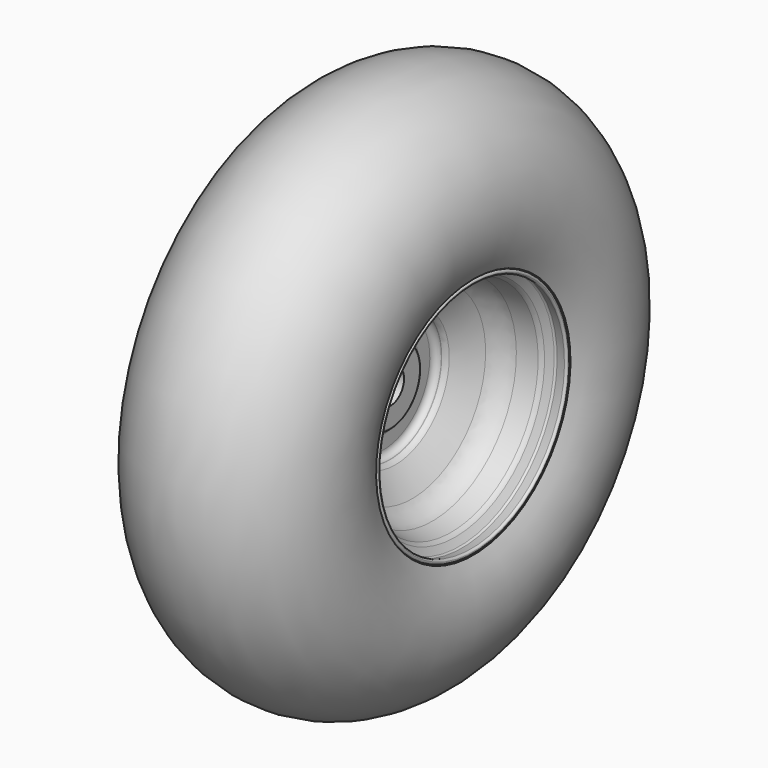
from build123d import *

# Parameters (mm, degrees)
F2_R  = 15
F3_R  = 3
F5_R  = 5
F6_R  = 15
F7_R  = 10
F8_R  = 3
F9_R  = 0.99999
F10_R = 1


# Not quite as in the source:
# - a fillet or chamfer that OpenCascade refuses, or shapes differently, is made with other operations: its cross-section is extruded or revolved along the edge and cut away or added
# - a fillet or chamfer is up to 0.001 mm smaller than in the source, because OpenCascade refuses the exact size


with BuildPart() as f1:
    # F0 (on Front) → F1 (revolve)
    with BuildSketch(Plane.XZ):
        Polygon((-55, 7.9375), (0, 7.9375), (0, 17.9375), (-3.4099393524, 17.9375), (-3.4099393524, 30.2716810256), (1.3420858886, 30.2716810256), (13.6318095028, 47.9688830674), (29.6903830022, 51.0822795331), (32.7981238869, 55.8634183106), (38.7093649285, 54.3856122498), (39.1944348812, 56.3258975744), (31.8988867003, 58.1497794366), (28.4762072553, 52.884119903), (12.4528761376, 49.7775561429), (0.2960184428, 32.2716810256), (-5.4099393524, 32.2716810256), (-5.4099393524, 17.9375), (-9.8811367593, 17.9375), (-5.8835780754, 22.3348141701), (-5.8835780754, 33.0104142308), (-12.7767843909, 37.2448114144), (-21.0078078969, 49.1898350166), (-37.3222876752, 51.9089149797), (-41.134234356, 58.0280866921), (-46.044562012, 58.0280866921), (-46.044562012, 56.0280866921), (-42.2446578741, 56.0280866921), (-38.5421812534, 50.0846430659), (-22.1733525395, 47.3565049469), (-14.1838043928, 35.7619151473), (-7.363458164, 31.5722748637), (-7.363458164, 23.6801598221), (-10.2864634246, 20.4648543149), (-20.127248019, 20.4648543149), (-20.127248019, 17.9375), (-55, 17.9375), align=None)
    revolve(axis=Axis((6.5463334322, 0, 0), (-1, 0, 0)))

    # F2
    f2_edges = [f1.edges().sort_by_distance(p)[0] for p in [
        (13.63181, 0, -47.968883),
    ]]
    fillet(f2_edges, radius=F2_R)

    # F3
    f3_edges = [f1.edges().sort_by_distance(p)[0] for p in [
        (-3.409939, 0, -30.271681),
        (1.342086, 0, -30.271681),
        (-3.409939, 0, -17.9375),
        (29.690383, 0, -51.08228),
    ]]
    fillet(f3_edges, radius=F3_R)

    # F4: fillet of radius 1 on 3 edges, made by hand

    # F4_s1 → F4_t2 (revolve)
    with BuildSketch(Plane.XZ):
        with BuildLine():
            ThreePointArc((32.4092989182, 55.265226182), (32.8817291061, 55.6508473382), (33.4902774565, 55.6903804099))
            Line((33.4902774565, 55.6903804099), (32.7981238869, 55.8634183106))
            Line((32.7981238869, 55.8634183106), (32.4092989182, 55.265226182))
        make_face()
    revolve(axis=Axis((32.7981238869, 0, 0), (-1, 0, 0)))

    # F4_s3 → F4_t4 (revolve, cut)
    with BuildSketch(Plane.XZ):
        with BuildLine():
            ThreePointArc((37.7392222662, 54.6281472261), (38.4962535713, 54.7407973068), (38.9518999049, 55.3557549121))
            Line((38.9518999049, 55.3557549121), (38.7093649285, 54.3856122498))
            Line((38.7093649285, 54.3856122498), (37.7392222662, 54.6281472261))
        make_face()
    revolve(axis=Axis((38.7093649285, 0, 0), (-1, 0, 0)), mode=Mode.SUBTRACT)

    # F4_s5 → F4_t6 (revolve, cut)
    with BuildSketch(Plane.XZ):
        with BuildLine():
            ThreePointArc((38.9518999049, 55.3557549121), (38.8392498242, 56.1127862172), (38.2242922189, 56.5684325508))
            Line((38.2242922189, 56.5684325508), (39.1944348812, 56.3258975744))
            Line((39.1944348812, 56.3258975744), (38.9518999049, 55.3557549121))
        make_face()
    revolve(axis=Axis((39.1944348812, 0, 0), (-1, 0, 0)), mode=Mode.SUBTRACT)

    # F5
    f5_edges = [f1.edges().sort_by_distance(p)[0] for p in [
        (28.476207, 0, -52.88412),
        (12.452876, 0, -49.777556),
        (31.898887, 0, -58.149779),
        (-37.322288, 0, -51.908915),
        (-41.134234, 0, -58.028087),
        (-21.007808, 0, -49.189835),
        (-12.776784, 0, -37.244811),
        (-16.892296, 0, 43.217323),
        (0.296018, 0, -32.271681),
    ]]
    fillet(f5_edges, radius=F5_R)

    # F6
    f6_edges = [f1.edges().sort_by_distance(p)[0] for p in [
        (-22.173353, 0, -47.356505),
    ]]
    fillet(f6_edges, radius=F6_R)

    # F7
    f7_edges = [f1.edges().sort_by_distance(p)[0] for p in [
        (-18.5634, 0, -42.117671),
        (-14.183804, 0, -35.761915),
    ]]
    fillet(f7_edges, radius=F7_R)

    # F8
    f8_edges = [f1.edges().sort_by_distance(p)[0] for p in [
        (-38.542181, 0, -50.084643),
        (-42.244658, 0, -56.028087),
    ]]
    fillet(f8_edges, radius=F8_R)

    # F9 (radius 1 in the source; OpenCascade refuses exactly that, so slightly less here)
    f9_edges = [f1.edges().sort_by_distance(p)[0] for p in [
        (-46.044562, 0, -58.028087),
        (-46.044562, 0, -56.028087),
    ]]
    fillet(f9_edges, radius=F9_R)

    # F10
    f10_edges = [f1.edges().sort_by_distance(p)[0] for p in [
        (-55, 0, -17.9375),
        (0, 0, -17.9375),
    ]]
    fillet(f10_edges, radius=F10_R)


with BuildPart() as f12:
    # F11 (on Front) → F12 (revolve)
    with BuildSketch(Plane.XZ):
        with BuildLine():
            Line((38.2242922189, 56.5684325508), (38.7676979443, 56.8790051404))
            ThreePointArc((38.7676979443, 56.8790051404), (-1.9823274862, 126.9890970924), (-45.6984266374, 58.689080686))
            Line((-45.6984266374, 58.689080686), (-45.044562012, 58.0280866921))
            Line((-45.044562012, 58.0280866921), (-43.9102931513, 58.0280866921))
            ThreePointArc((-43.9102931513, 58.0280866921), (-41.4832270066, 57.399510937), (-39.6663988357, 55.6718266638))
            Line((-39.6663988357, 55.6718266638), (-38.5164480451, 53.8258547922))
            Line((-38.5164480451, 53.8258547922), (-33.0451540649, 58.5665740073))
            Line((-33.0451540649, 58.5665740073), (-36.1832785465, 62.1883032864))
            Line((-36.1832785465, 62.1883032864), (-41.0874944461, 63.7939320093))
            ThreePointArc((-41.0874944461, 63.7939320093), (-2.7023885343, 120.6976847932), (34.856610424, 63.2453129188))
            Line((34.856610424, 63.2453129188), (32.0315919816, 61.3080300391))
            Line((32.0315919816, 61.3080300391), (23.1617614627, 57.9845495522))
            Line((23.1617614627, 57.9845495522), (26.3924346364, 52.4801232275))
            ThreePointArc((26.3924346364, 52.4801232275), (28.2348643151, 53.2422735342), (29.6329856976, 54.663778656))
            Line((29.6329856976, 54.663778656), (29.9547618573, 55.1588187934))
            ThreePointArc((29.9547618573, 55.1588187934), (32.3169127965, 57.0869245744), (35.3596545484, 57.2845899332))
            Line((35.3596545484, 57.2845899332), (38.2242922189, 56.5684325508))
        make_face()
    revolve(axis=Axis((-10.1076848805, 0, 0), (1, 0, 0)))


solid = Compound([f1.part, f12.part])
